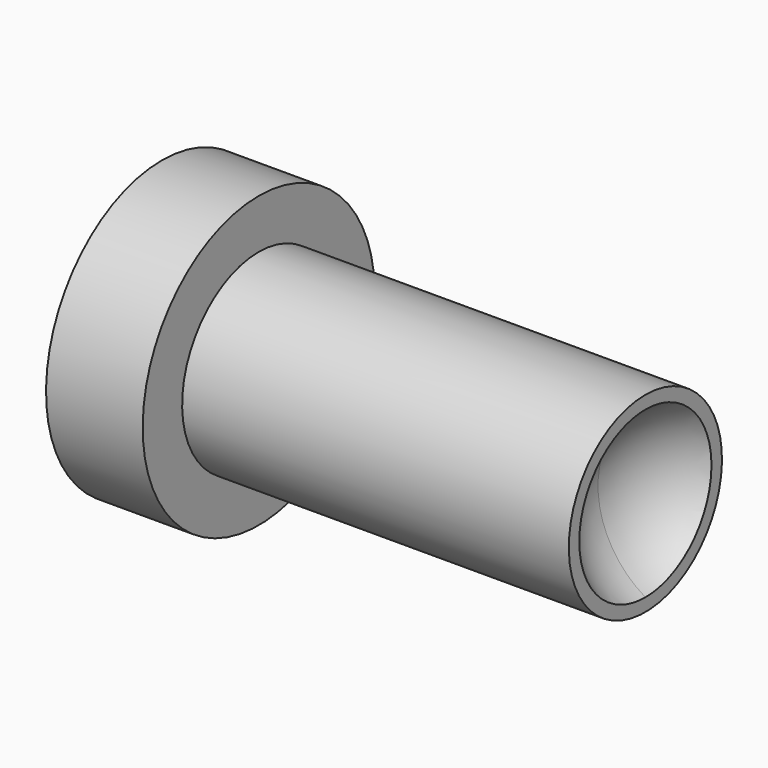
from build123d import *
from build123d import SkipClean  # not in build123d's __all__


with BuildPart() as f1:
    # F0 (on Front) → F1 (revolve)
    with BuildSketch(Plane.XZ):
        Polygon((0, 19.05), (-12.7, 19.05), (-12.7, 0), (0, 0), (50.8, 0), (50.8, 12.573), (0, 12.573), align=None)
    revolve(axis=Axis((25.4, 0, 0), (1, 0, 0)))

    # F2 (on Front) → F3 (revolve, cut)
    with BuildSketch(Plane.XZ):
        with BuildLine():
            Line((57.15, 0), (57.15, 12.573))
            ThreePointArc((57.15, 12.573), (44.577, 0), (57.15, -12.573))
            Line((57.15, -12.573), (57.15, 0))
        make_face()
    with SkipClean():  # cleaning this boolean's faces spoils the solid; the shape is the same uncleaned
        revolve(axis=Axis((57.15, 0, 0), (0, 0, 1)), mode=Mode.SUBTRACT)


solid = f1.part
